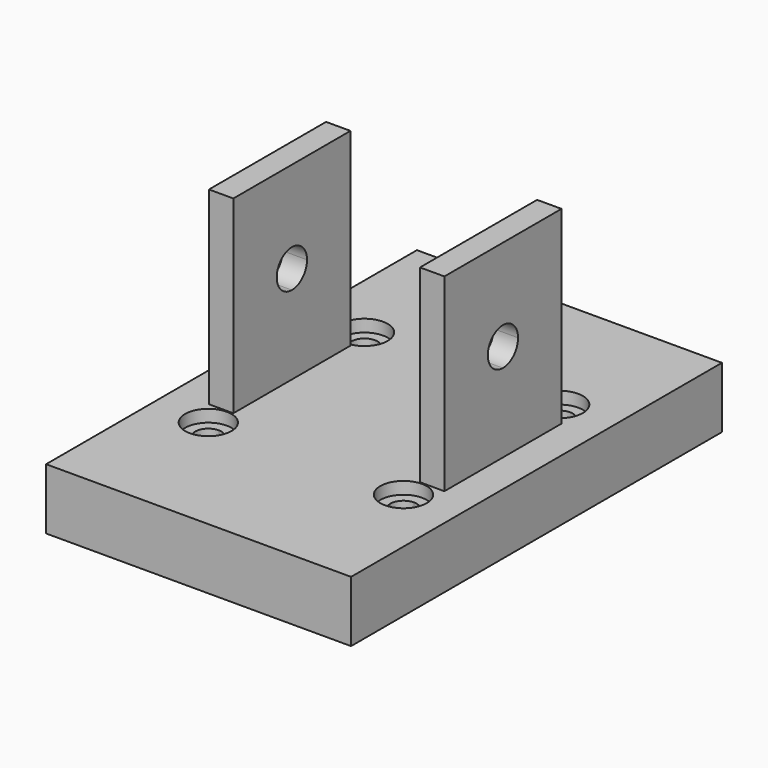
from build123d import *

# Parameters (mm, degrees)
F0_W     = 25
F0_H     = 38
F1_DEPTH = 5
F3_DEPTH = 5
F5_DEPTH = 15.5
F7_DEPTH = 25
F8_R     = 1.9
F9_DEPTH = 1


# Not quite as in the source:
# - a feature names something its author has since deleted; it is built from what else it names


with BuildPart() as f1:
    # F0 (on Top) → F1 (new body)
    with BuildSketch(Plane.XY):
        with Locations((-5.6626851261, 7.8445598302)):
            Rectangle(F0_W, F0_H)
    extrude(amount=F1_DEPTH)

    # F2 (on face) → F3 (cut)
    with BuildSketch(Plane.XY.offset(5)):
        with BuildLine():
            Line((-13.6626851261, 15.8445598302), (-12.5876851261, 15.8445598302))
            ThreePointArc((-12.5876851261, 15.8445598302), (-14.4228249158, 16.60469962), (-13.6626851261, 14.7695598302))
            Line((-13.6626851261, 14.7695598302), (-13.6626851261, 15.8445598302))
        make_face()
        with BuildLine():
            ThreePointArc((-13.6626851261, 14.7695598302), (-12.9025453363, 15.0844200404), (-12.5876851261, 15.8445598302))
            Line((-12.5876851261, 15.8445598302), (-13.6626851261, 15.8445598302))
            Line((-13.6626851261, 15.8445598302), (-13.6626851261, 14.7695598302))
        make_face()
        with BuildLine():
            Line((2.3373148739, 15.8445598302), (1.2623148739, 15.8445598302))
            ThreePointArc((1.2623148739, 15.8445598302), (1.5771750842, 15.0844200404), (2.3373148739, 14.7695598302))
            Line((2.3373148739, 14.7695598302), (2.3373148739, 15.8445598302))
        make_face()
        with BuildLine():
            ThreePointArc((3.4123148739, 15.8445598302), (2.3373148739, 16.9195598302), (1.2623148739, 15.8445598302))
            Line((1.2623148739, 15.8445598302), (2.3373148739, 15.8445598302))
            Line((2.3373148739, 15.8445598302), (2.3373148739, 14.7695598302))
            ThreePointArc((2.3373148739, 14.7695598302), (3.0974546637, 15.0844200404), (3.4123148739, 15.8445598302))
        make_face()
        with BuildLine():
            Line((-13.6626851261, -0.1554401698), (-13.6626851261, 0.9195598302))
            ThreePointArc((-13.6626851261, 0.9195598302), (-14.4228249158, -0.9155799596), (-12.5876851261, -0.1554401698))
            Line((-12.5876851261, -0.1554401698), (-13.6626851261, -0.1554401698))
        make_face()
        with BuildLine():
            ThreePointArc((-12.5876851261, -0.1554401698), (-12.9025453363, 0.60469962), (-13.6626851261, 0.9195598302))
            Line((-13.6626851261, 0.9195598302), (-13.6626851261, -0.1554401698))
            Line((-13.6626851261, -0.1554401698), (-12.5876851261, -0.1554401698))
        make_face()
        with BuildLine():
            Line((2.3373148739, -0.1554401698), (2.3373148739, 0.9195598302))
            ThreePointArc((2.3373148739, 0.9195598302), (1.5771750842, 0.60469962), (1.2623148739, -0.1554401698))
            Line((1.2623148739, -0.1554401698), (2.3373148739, -0.1554401698))
        make_face()
        with BuildLine():
            ThreePointArc((3.4123148739, -0.1554401698), (3.0974546637, 0.60469962), (2.3373148739, 0.9195598302))
            Line((2.3373148739, 0.9195598302), (2.3373148739, -0.1554401698))
            Line((2.3373148739, -0.1554401698), (1.2623148739, -0.1554401698))
            ThreePointArc((1.2623148739, -0.1554401698), (2.3373148739, -1.2304401698), (3.4123148739, -0.1554401698))
        make_face()
    extrude(amount=-F3_DEPTH, mode=Mode.SUBTRACT)

    # F4 (on face) → F5 (join)
    with BuildSketch(Plane.XY.offset(5)):
        Polygon((-15.2126851261, 13.8445598302), (-15.2126851261, 1.8445598302), (-14.2126851261, 1.8445598302), (-13.2126851261, 1.8445598302), (-13.2126851261, 13.8445598302), (-14.2126851261, 13.8445598302), align=None)
        Polygon((4.0873148739, 13.8445598302), (3.0873148739, 13.8445598302), (2.0873148739, 13.8445598302), (2.0873148739, 1.8445598302), (4.0873148739, 1.8445598302), align=None)
    extrude(amount=F5_DEPTH)

    # F6 (on face) → F7 (cut)
    with BuildSketch(Plane.YZ.offset(4.0873148739)):
        with BuildLine():
            Line((7.8445598302, 11.45), (7.8445598302, 14.55))
            ThreePointArc((7.8445598302, 14.55), (6.2945598302, 13), (7.8445598302, 11.45))
        make_face()
        with BuildLine():
            ThreePointArc((7.8445598302, 11.45), (8.9405753411, 11.9039844892), (9.3945598302, 13))
            ThreePointArc((9.3945598302, 13), (8.9405753411, 14.0960155108), (7.8445598302, 14.55))
            Line((7.8445598302, 14.55), (7.8445598302, 11.45))
        make_face()
    extrude(amount=-F7_DEPTH, mode=Mode.SUBTRACT)

    # F8 (on face) → F9 (cut)
    with BuildSketch(Plane.XY.offset(5)):
        with Locations((-13.6626851261, 15.8445598302)):
            Circle(F8_R)
        with Locations((2.3373148739, 15.8445598302)):
            Circle(F8_R)
        with Locations((2.3373148739, -0.1554401698)):
            Circle(F8_R)
        with Locations((-13.6626851261, -0.1554401698)):
            Circle(F8_R)
    extrude(amount=-F9_DEPTH, mode=Mode.SUBTRACT)


solid = f1.part
